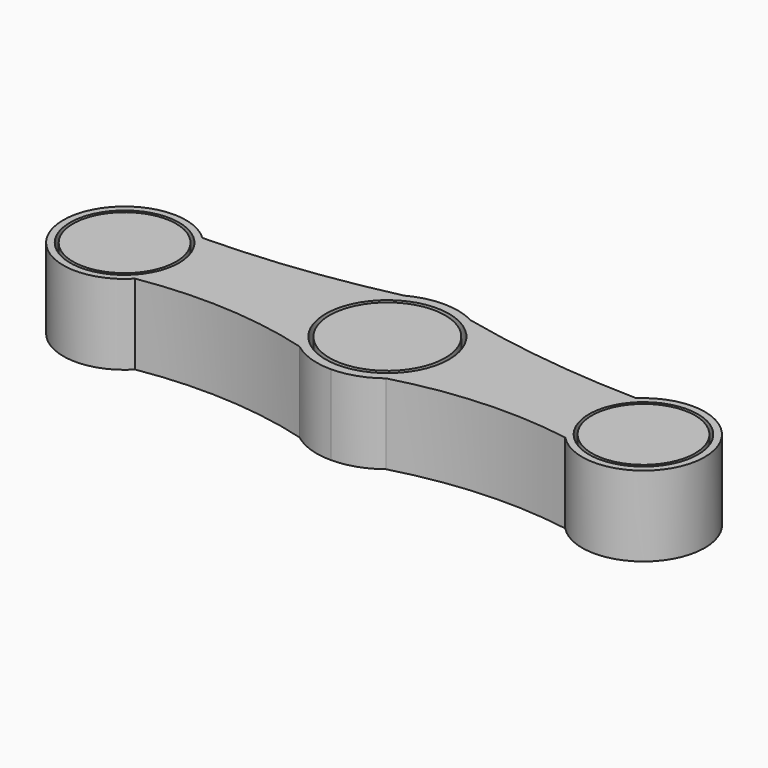
from build123d import *

# Parameters (mm, degrees)
F0_R     = 5.1963002221
F0_R_2   = 5.8800950513
F1_DEPTH = 7.62
F0_R_3   = 5.5044911899
F0_R_4   = 4.9042601262


# Not quite as in the source:
# - a feature names something its author has since deleted; it is built from what else it names


with BuildPart() as f1:
    # F0 (on Top) → F1 (new body)
    with BuildSketch(Plane.XY):
        with BuildLine():
            ThreePointArc((-3.1544311234, 5.9388807954), (-1.573442924, 6.3166135062), (0, 6.7246368537))
            ThreePointArc((0, 6.7246368537), (-1.6254113553, 6.5252416614), (-3.1544311234, 5.9388807954))
        make_face()
        with BuildLine():
            ThreePointArc((0, 6.7246368537), (1.573442924, 6.3166135062), (3.1544311234, 5.9388807954))
            ThreePointArc((3.1544311234, 5.9388807954), (1.6254113553, 6.5252416614), (0, 6.7246368537))
        make_face()
        with BuildLine():
            ThreePointArc((0, -6.7246368537), (2.1790400303, -6.3618020529), (4.1229353018, -5.3124519114))
            ThreePointArc((4.1229353018, -5.3124519114), (2.0411071075, -5.9591008914), (0, -6.7246368537))
        make_face()
        with BuildLine():
            ThreePointArc((-4.1229353018, -5.3124519114), (-2.1790400303, -6.3618020529), (0, -6.7246368537))
            ThreePointArc((0, -6.7246368537), (-2.0411071075, -5.9591008914), (-4.1229353018, -5.3124519114))
        make_face()
        with BuildLine():
            ThreePointArc((-4.1229353018, -5.3124519114), (-6.6998610017, 0.5767177582), (-3.1544311234, 5.9388807954))
            ThreePointArc((-3.1544311234, 5.9388807954), (-11.8536034806, 4.4211029843), (-20.6635650247, 3.8179224357))
            ThreePointArc((-20.6635650247, 3.8179224357), (-30.545156174, -0.5250277146), (-20.481782034, -4.4283033349))
            ThreePointArc((-20.481782034, -4.4283033349), (-12.2539035705, -3.9738433369), (-4.1229353018, -5.3124519114))
        make_face()
        with Locations((-24.706566421, -0.3963195836)):
            Circle(F0_R, mode=Mode.SUBTRACT)
        with BuildLine():
            ThreePointArc((3.1544311234, 5.9388807954), (5.7633820192, 3.4647032362), (6.7246368537, 0))
            ThreePointArc((6.7246368537, 0), (6.0392873541, -2.9576593903), (4.1229353018, -5.3124519114))
            ThreePointArc((4.1229353018, -5.3124519114), (12.2539035705, -3.9738433369), (20.481782034, -4.4283033349))
            ThreePointArc((20.481782034, -4.4283033349), (30.545156174, -0.5250277146), (20.6635650247, 3.8179224357))
            ThreePointArc((20.6635650247, 3.8179224357), (11.8536034806, 4.4211029843), (3.1544311234, 5.9388807954))
        make_face()
        with Locations((24.706566421, -0.3963195836)):
            Circle(F0_R, mode=Mode.SUBTRACT)
        with BuildLine():
            ThreePointArc((4.1229353018, -5.3124519114), (6.0392873541, -2.9576593903), (6.7246368537, 0))
            ThreePointArc((6.7246368537, 0), (5.7633820192, 3.4647032362), (3.1544311234, 5.9388807954))
            ThreePointArc((3.1544311234, 5.9388807954), (1.573442924, 6.3166135062), (0, 6.7246368537))
            ThreePointArc((0, 6.7246368537), (-1.573442924, 6.3166135062), (-3.1544311234, 5.9388807954))
            ThreePointArc((-3.1544311234, 5.9388807954), (-6.6998610017, 0.5767177582), (-4.1229353018, -5.3124519114))
            ThreePointArc((-4.1229353018, -5.3124519114), (-2.0411071075, -5.9591008914), (0, -6.7246368537))
            ThreePointArc((0, -6.7246368537), (2.0411071075, -5.9591008914), (4.1229353018, -5.3124519114))
        make_face()
        Circle(F0_R_2, mode=Mode.SUBTRACT)
    extrude(amount=F1_DEPTH)


with BuildPart() as f1b:
    # F0 (on Top) → F1, piece 2 (new body)
    with BuildSketch(Plane.XY):
        Circle(F0_R_3)
    extrude(amount=F1_DEPTH)


with BuildPart() as f1c:
    # F0 (on Top) → F1, piece 3 (new body)
    with BuildSketch(Plane.XY):
        with Locations((24.706566421, -0.3963195836)):
            Circle(F0_R_4)
    extrude(amount=F1_DEPTH)


with BuildPart() as f1d:
    # F0 (on Top) → F1, piece 4 (new body)
    with BuildSketch(Plane.XY):
        with Locations((-24.706566421, -0.3963195836)):
            Circle(F0_R_4)
    extrude(amount=F1_DEPTH)


solid = Compound([f1.part, f1b.part, f1c.part, f1d.part])
